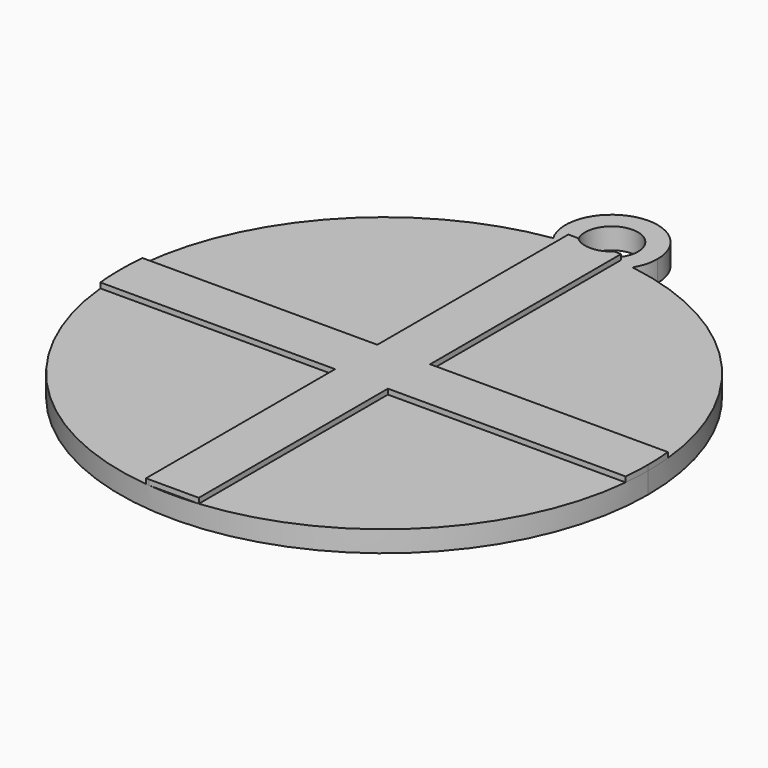
from build123d import *

# Parameters (mm, degrees)
F1_DEPTH = 2
F2_W     = 5
F2_H     = 5
F3_DEPTH = 0.5
F4_D     = 5


# Not quite as in the source:
# - a feature names something its author has since deleted; it is built from what else it names


with BuildPart() as f1:
    # F0 (on Top) → F1 (new body)
    with BuildSketch(Plane.XY):
        with BuildLine():
            ThreePointArc((-3.7594057481, 24.7157210783), (0, 25), (3.7594057481, 24.7157210783))
            ThreePointArc((3.7594057481, 24.7157210783), (4.209761495, 25.7828537011), (4.3634907466, 26.9308779389))
            ThreePointArc((4.3634907466, 26.9308779389), (-1.1480242378, 31.1406394339), (-3.7594057481, 24.7157210783))
        make_face()
        with BuildLine():
            ThreePointArc((-3.7594057481, 24.7157210783), (0, 22.5673871923), (3.7594057481, 24.7157210783))
            ThreePointArc((3.7594057481, 24.7157210783), (0, 25), (-3.7594057481, 24.7157210783))
        make_face()
        with BuildLine():
            ThreePointArc((-3.7594057481, 24.7157210783), (-16.2943986741, -18.9602893399), (25, 0))
            ThreePointArc((25, 0), (18.9602893399, 16.2943986741), (3.7594057481, 24.7157210783))
            ThreePointArc((3.7594057481, 24.7157210783), (0, 22.5673871923), (-3.7594057481, 24.7157210783))
        make_face()
    extrude(amount=F1_DEPTH)

    # F2 (on face) → F3 (join)
    with BuildSketch(Plane.XY.offset(2)):
        Polygon((-2.640592387, 25.1115851104), (-2.640592387, 2.5), (2.359407613, 2.5), (2.359407613, 25.1115851104), (-0.140592387, 25.1115851104), align=None)
        with BuildLine():
            Line((-2.640592387, 2.5), (-24.8746859277, 2.5))
            ThreePointArc((-24.8746859277, 2.5), (-24.9686518278, 1.2515693765), (-25, 0))
            ThreePointArc((-25, 0), (-24.9686518278, -1.2515693765), (-24.8746859277, -2.5))
            Line((-24.8746859277, -2.5), (-2.640592387, -2.5))
            Line((-2.640592387, -2.5), (-2.640592387, 2.5))
        make_face()
        with Locations((-0.140592387, 0)):
            Rectangle(F2_W, F2_H)
        with BuildLine():
            Line((24.8746859277, 2.5), (2.359407613, 2.5))
            Line((2.359407613, 2.5), (2.359407613, -2.5))
            Line((2.359407613, -2.5), (24.8746859277, -2.5))
            ThreePointArc((24.8746859277, -2.5), (24.9686518278, -1.2515693765), (25, 0))
            ThreePointArc((25, 0), (24.9686518278, 1.2515693765), (24.8746859277, 2.5))
        make_face()
        with BuildLine():
            Line((2.359407613, -2.5), (-2.640592387, -2.5))
            Line((-2.640592387, -2.5), (-2.640592387, -24.8601543005))
            ThreePointArc((-2.640592387, -24.8601543005), (-2.5000399327, -24.8746819142), (-2.359407613, -24.8884148896))
            Line((-2.359407613, -24.8884148896), (-0.140592387, -24.8884148896))
            Line((-0.140592387, -24.8884148896), (2.359407613, -24.8884148896))
            Line((2.359407613, -24.8884148896), (2.359407613, -2.5))
        make_face()
    extrude(amount=F3_DEPTH)

    # F4 (through all)
    with Locations(Plane(origin=(0, 0, 0), x_dir=(1, 0, 0), z_dir=(0, 0, -1))):
        with Locations((0, -26.9308779389)):
            Hole(F4_D / 2)


solid = f1.part
